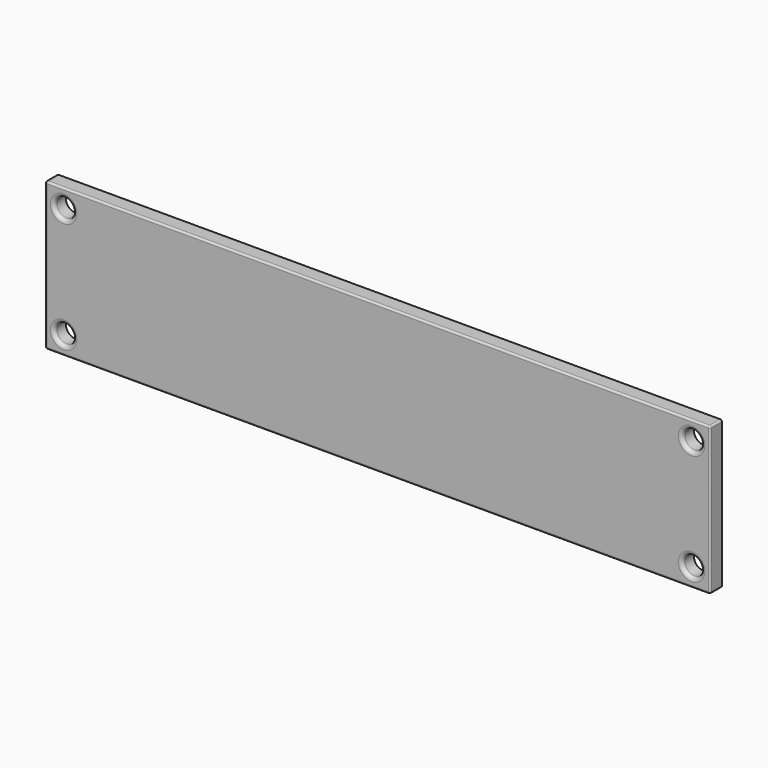
from build123d import *

# Parameters (mm, degrees)
F0_W         = 180
F0_H         = 40
F0_R         = 2.5751263091
F1_DEPTH     = 4
F2_R         = 1
F3_R         = 0.5
F4_TEXT_SIZE = 10.8126372698
F5_DEPTH     = 1


# Not quite as in the source:
# - a feature names something its author has since deleted; it is built from what else it names
# - Text() gives the source's letters only with a copy of the font that has no kerning and outlines rounded to 1/6400 em; it was checked with that copy


with BuildPart() as f1:
    # F0 (on Front) → F1 (new body)
    with BuildSketch(Plane.XZ):
        Rectangle(F0_W, F0_H)
        with Locations((-85, -15)):
            Circle(F0_R, mode=Mode.SUBTRACT)
        with Locations((85, -15)):
            Circle(F0_R, mode=Mode.SUBTRACT)
        with Locations((-85, 15)):
            Circle(F0_R, mode=Mode.SUBTRACT)
        with Locations((85, 15)):
            Circle(F0_R, mode=Mode.SUBTRACT)
    extrude(amount=F1_DEPTH)

    # F2
    f2_edges = [f1.edges().sort_by_distance(p)[0] for p in [
        (-87.575126, -4, 15),
        (-87.575126, -4, -15),
        (82.424874, -4, 15),
        (82.424874, -4, -15),
    ]]
    fillet(f2_edges, radius=F2_R)

    # F3
    f3_edges = [f1.edges().sort_by_distance(p)[0] for p in [
        (0, -4, 20),
        (-90, -4, 0),
        (0, -4, -20),
        (90, -4, 0),
        (-90, -2, 20),
        (-90, -2, -20),
        (90, -2, 20),
        (90, -2, -20),
    ]]
    fillet(f3_edges, radius=F3_R)

    # F4 (on face) → F5 (join)
    with BuildSketch(Plane(origin=(0, 0, 0), x_dir=(-1, 0, 0), z_dir=(0, 1, 0))):
        with Locations((-64.729437232, -1.0298250451)):
            Text('Virage Body', F4_TEXT_SIZE, font='Open Sans', text_align=(TextAlign.LEFT, TextAlign.BOTTOM))
    extrude(amount=F5_DEPTH)

    # F6: F1 across plane


with BuildPart() as f1_1:
    add(f1.part)
    add(f1.part.mirror(Plane.YZ))


solid = f1_1.part
